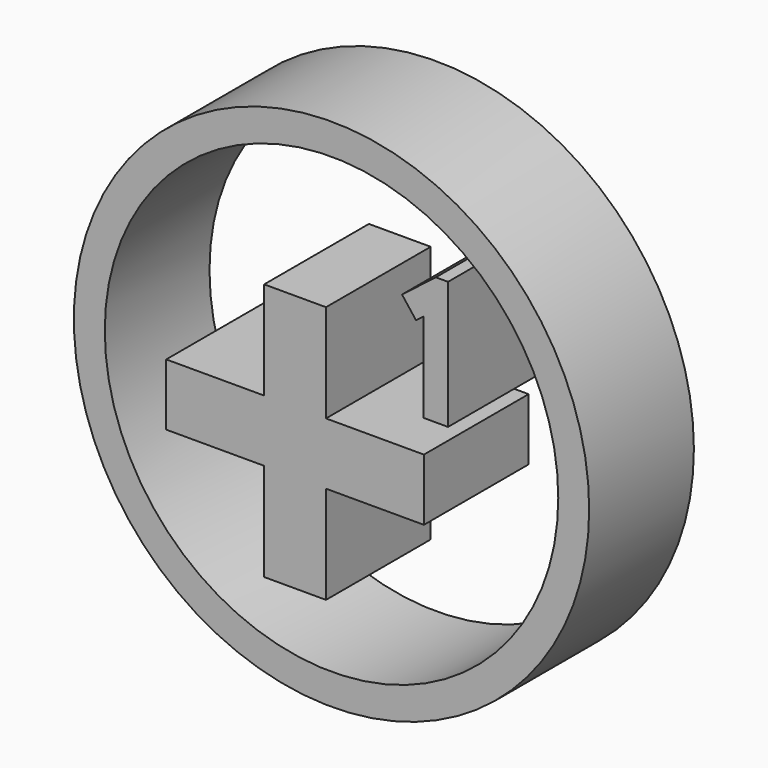
from build123d import *

# Parameters (mm, degrees)
F0_R         = 50
F0_R_2       = 44
F1_DEPTH     = 25.4
F0_W         = 12
F0_H         = 12
F0_W_2       = 19
F0_H_2       = 19
F0_TEXT_SIZE = 34.7222222222
F2_DEPTH     = 25.4
F4_DEPTH     = 14.478


# Not quite as in the source:
# - a feature names something its author has since deleted; it is built from what else it names
# - Text() gives the source's letters only with a copy of the font that has no kerning and outlines rounded to 1/6400 em; it was checked with that copy


with BuildPart() as f1:
    # F0 (on Front) → F1 (new body)
    with BuildSketch(Plane.XZ):
        Circle(F0_R)
        Circle(F0_R_2, mode=Mode.SUBTRACT)
    extrude(amount=F1_DEPTH)


with BuildPart() as f2:
    # F0 (on Front) → F2 (new body)
    with BuildSketch(Plane.XZ):
        with Locations((-7.0710678119, -7.0710678119)):
            Rectangle(F0_W, F0_H)
        with Locations((-22.5710678119, -7.0710678119)):
            Rectangle(F0_W_2, F0_H)
        with Locations((8.4289321881, -7.0710678119)):
            Rectangle(F0_W_2, F0_H)
        with Locations((-7.0710678119, -22.5710678119)):
            Rectangle(F0_W, F0_H_2)
        with Locations((-7.0710678119, 8.4289321881)):
            Rectangle(F0_W, F0_H_2)
        with Locations((10.4917971338, 5.1776695297)):
            Text('1', F0_TEXT_SIZE, font='Open Sans', text_align=(TextAlign.LEFT, TextAlign.BOTTOM))
    extrude(amount=F2_DEPTH)

    # F3 (on face) → F4 (join)
    with BuildSketch(Plane.XZ.offset(25.4)):
        Polygon((17.8667971338, 5.1776695297), (19.8667971338, 5.1776695297), (22.6120228283, 5.1776695297), (20.6548700741, 28.6309396105), (18.0274471641, 25.3570372825), (17.8667971338, 25.1568591893), (17.8667971338, 22.5149448376), align=None)
        Polygon((16.3965137036, 21.3791921879), (17.8667971338, 22.5149448376), (17.8667971338, 25.1568591893), (18.0274471641, 25.3570372825), (15.1738717866, 22.9619577241), align=None)
    extrude(amount=-F4_DEPTH)


solid = Compound([f1.part, f2.part])
